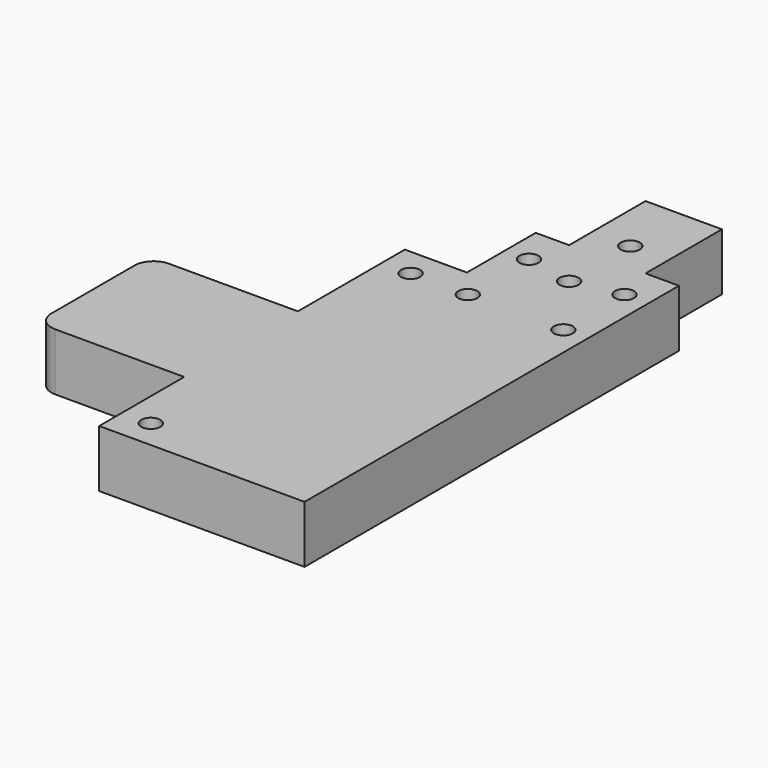
from build123d import *

# Parameters (mm, degrees)
F0_R     = 3.175
F1_DEPTH = 19.05
F2_R     = 3.175
F3_DEPTH = 25.4
F4_R     = 6.35


with BuildPart() as f1:
    # F0 (on Top) → F1 (new body)
    with BuildSketch(Plane.XY):
        Polygon((21.1725122346, -375.6896027952), (21.1725122346, -220.1146027952), (10.0600122346, -220.1146027952), (10.0600122346, -188.3646027952), (-15.3399877654, -188.3646027952), (-15.3399877654, -210.5896027952), (-15.3399877654, -220.1146027952), (-26.4524877654, -220.1146027952), (-26.4524877654, -248.6896067858), (-47.0899877654, -248.6896067858), (-47.0899877654, -293.1396027952), (-96.3024877654, -293.1396027952), (-96.3024877654, -314.9836027952), (-96.3024877654, -340.3836027952), (-47.0899877654, -340.3836027952), (-47.0899877654, -375.6896027952), (-26.4524877654, -375.6896027952), (-13.7524877654, -375.6896027952), align=None)
        with Locations((-37.5649877654, -366.1646027952)):
            Circle(F0_R, mode=Mode.SUBTRACT)
        with Locations((-37.5649877654, -258.2146027952)):
            Circle(F0_R, mode=Mode.SUBTRACT)
        with Locations((-2.6399877654, -235.9896027952)):
            Circle(F0_R, mode=Mode.SUBTRACT)
        with Locations((-2.6399877654, -210.5896027952)):
            Circle(F0_R, mode=Mode.SUBTRACT)
    extrude(amount=F1_DEPTH)

    # F2 (on face) → F3 (cut)
    with BuildSketch(Plane.XY.offset(19.05)):
        with Locations((-18.5149877654, -232.8146027952)):
            Circle(F2_R)
        with Locations((13.2350122346, -232.8146027952)):
            Circle(F2_R)
        with Locations((13.2350122346, -258.2146027952)):
            Circle(F2_R)
        with Locations((-18.5149877654, -258.2146027952)):
            Circle(F2_R)
    extrude(amount=-F3_DEPTH, mode=Mode.SUBTRACT)

    # F4
    f4_edges = [f1.edges().sort_by_distance(p)[0] for p in [
        (-96.302488, -340.383603, 9.525),
        (-96.302488, -293.139603, 9.525),
    ]]
    fillet(f4_edges, radius=F4_R)


solid = f1.part
